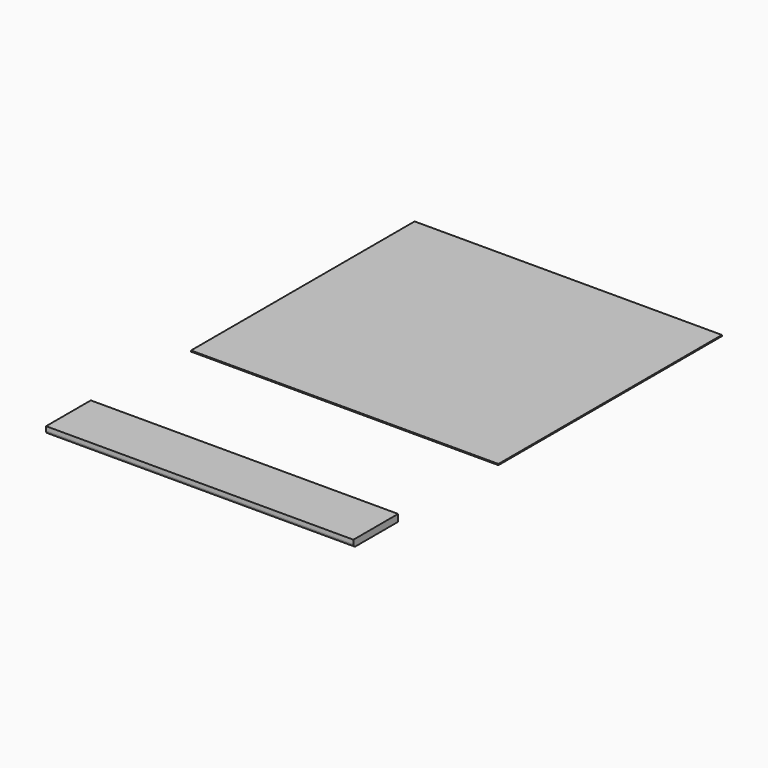
from build123d import *

# Parameters (mm, degrees)
F0_W     = 558.8
F0_H     = 508
F1_DEPTH = 2.032
F2_W     = 558.8
F2_H     = 101.6
F3_DEPTH = 12.7
F4_R     = 5.08


# Not quite as in the source:
# - a length typed as a fraction of an inch, garbled in the dataset ("3 / 203.2 mm" for 3/8 in), is restored


with BuildPart() as f1:
    # F0 (on Top) → F1 (new body)
    with BuildSketch(Plane.XY):
        Rectangle(F0_W, F0_H)
    extrude(amount=F1_DEPTH)


with BuildPart() as f3:
    # F2 (on face) → F3 (new body)
    with BuildSketch(Plane.XY.offset(2.032)):
        with Locations((0, -532.7320098877)):
            Rectangle(F2_W, F2_H)
    extrude(amount=F3_DEPTH)

    # F4
    f4_edges = [f3.edges().sort_by_distance(p)[0] for p in [
        (0, -583.53201, 2.032),
    ]]
    fillet(f4_edges, radius=F4_R)


solid = Compound([f1.part, f3.part])
